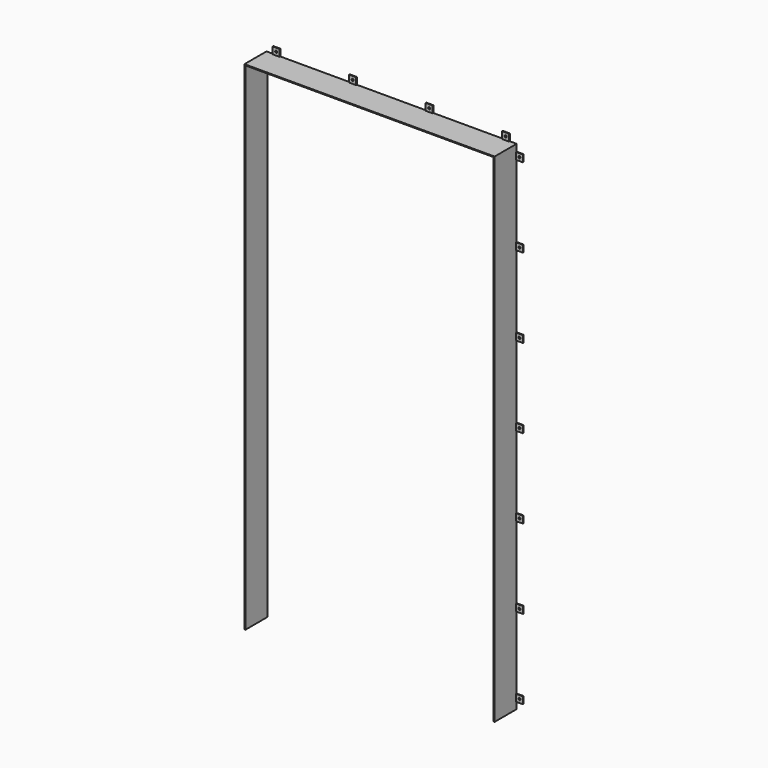
from build123d import *

# Parameters (mm, degrees)
F1_DEPTH = 101.6
F0_W     = 25.4
F0_H     = 25.4
F0_R     = 3.81
F2_DEPTH = 3.175


# Not quite as in the source:
# - a feature names something its author has since deleted; it is built from what else it names


with BuildPart() as f1:
    # F0 (on Front) → F1 (new body)
    with BuildSketch(Plane.XZ):
        Polygon((0, 25.4), (0, 0), (3.175, 0), (3.175, 1828.8), (917.575, 1828.8), (917.575, 0), (920.75, 0), (920.75, 25.4), (920.75, 50.8), (920.75, 318.0291666667), (920.75, 343.4291666667), (920.75, 610.6583333333), (920.75, 636.0583333333), (920.75, 903.2875), (920.75, 928.6875), (920.75, 1195.9166666667), (920.75, 1221.3166666667), (920.75, 1488.5458333333), (920.75, 1513.9458333333), (920.75, 1781.175), (920.75, 1806.575), (920.75, 1831.975), (895.35, 1831.975), (869.95, 1831.975), (613.8333333333, 1831.975), (588.4333333333, 1831.975), (332.3166666667, 1831.975), (306.9166666667, 1831.975), (50.8, 1831.975), (25.4, 1831.975), (0, 1831.975), (0, 1806.575), (0, 1781.175), (0, 1513.9458333333), (0, 1488.5458333333), (0, 1221.3166666667), (0, 1195.9166666667), (0, 928.6875), (0, 903.2875), (0, 636.0583333333), (0, 610.6583333333), (0, 343.4291666667), (0, 318.0291666667), (0, 50.8), align=None)
    extrude(amount=F1_DEPTH)

    # F0 (on Front) → F2 (join)
    with BuildSketch(Plane.XZ):
        with Locations((-12.7, 38.1)):
            Rectangle(F0_W, F0_H)
        with Locations((-12.7, 38.1)):
            Circle(F0_R, mode=Mode.SUBTRACT)
        with Locations((-12.7, 330.7291666667)):
            Rectangle(F0_W, F0_H)
        with Locations((-12.7, 330.7291666667)):
            Circle(F0_R, mode=Mode.SUBTRACT)
        with Locations((-12.7, 623.3583333333)):
            Rectangle(F0_W, F0_H)
        with Locations((-12.7, 623.3583333333)):
            Circle(F0_R, mode=Mode.SUBTRACT)
        with Locations((933.45, 38.1)):
            Rectangle(F0_W, F0_H)
        with Locations((933.45, 38.1)):
            Circle(F0_R, mode=Mode.SUBTRACT)
        with Locations((-12.7, 915.9875)):
            Rectangle(F0_W, F0_H)
        with Locations((-12.7, 915.9875)):
            Circle(F0_R, mode=Mode.SUBTRACT)
        with Locations((933.45, 330.7291666667)):
            Rectangle(F0_W, F0_H)
        with Locations((933.45, 330.7291666667)):
            Circle(F0_R, mode=Mode.SUBTRACT)
        with Locations((-12.7, 1208.6166666667)):
            Rectangle(F0_W, F0_H)
        with Locations((-12.7, 1208.6166666667)):
            Circle(F0_R, mode=Mode.SUBTRACT)
        with Locations((933.45, 623.3583333333)):
            Rectangle(F0_W, F0_H)
        with Locations((933.45, 623.3583333333)):
            Circle(F0_R, mode=Mode.SUBTRACT)
        with Locations((-12.7, 1501.2458333333)):
            Rectangle(F0_W, F0_H)
        with Locations((-12.7, 1501.2458333333)):
            Circle(F0_R, mode=Mode.SUBTRACT)
        with Locations((933.45, 915.9875)):
            Rectangle(F0_W, F0_H)
        with Locations((933.45, 915.9875)):
            Circle(F0_R, mode=Mode.SUBTRACT)
        with Locations((-12.7, 1793.875)):
            Rectangle(F0_W, F0_H)
        with Locations((-12.7, 1793.875)):
            Circle(F0_R, mode=Mode.SUBTRACT)
        with Locations((933.45, 1208.6166666667)):
            Rectangle(F0_W, F0_H)
        with Locations((933.45, 1208.6166666667)):
            Circle(F0_R, mode=Mode.SUBTRACT)
        with Locations((38.1, 1844.675)):
            Rectangle(F0_W, F0_H)
        with Locations((38.1, 1844.675)):
            Circle(F0_R, mode=Mode.SUBTRACT)
        with Locations((933.45, 1501.2458333333)):
            Rectangle(F0_W, F0_H)
        with Locations((933.45, 1501.2458333333)):
            Circle(F0_R, mode=Mode.SUBTRACT)
        with Locations((319.6166666667, 1844.675)):
            Rectangle(F0_W, F0_H)
        with Locations((319.6166666667, 1844.675)):
            Circle(F0_R, mode=Mode.SUBTRACT)
        with Locations((933.45, 1793.875)):
            Rectangle(F0_W, F0_H)
        with Locations((933.45, 1793.875)):
            Circle(F0_R, mode=Mode.SUBTRACT)
        with Locations((601.1333333333, 1844.675)):
            Rectangle(F0_W, F0_H)
        with Locations((601.1333333333, 1844.675)):
            Circle(F0_R, mode=Mode.SUBTRACT)
        with Locations((882.65, 1844.675)):
            Rectangle(F0_W, F0_H)
        with Locations((882.65, 1844.675)):
            Circle(F0_R, mode=Mode.SUBTRACT)
    extrude(amount=F2_DEPTH)


solid = f1.part
